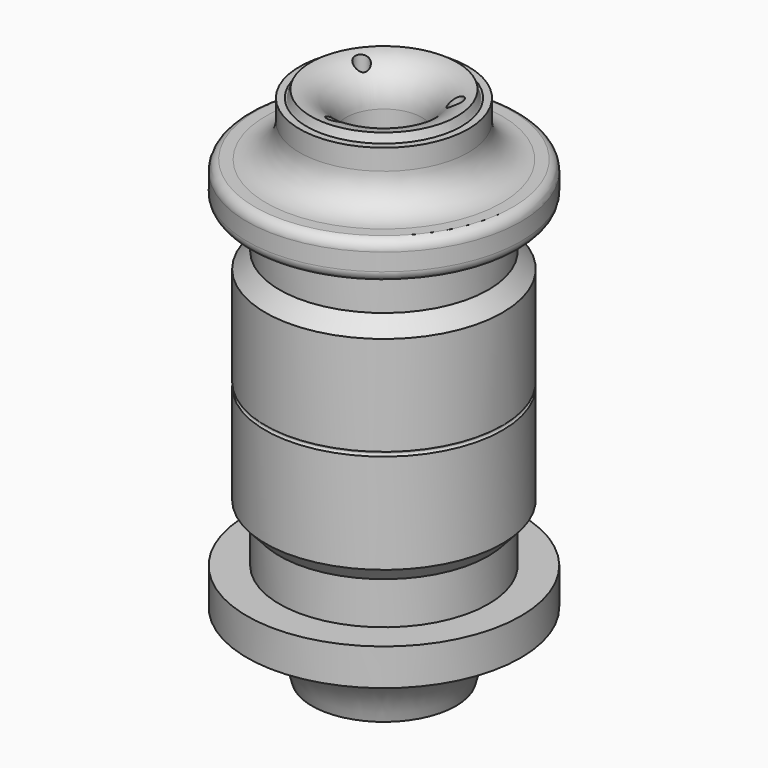
from build123d import *

# Parameters (mm, degrees)
F2_R     = 0.9926331533
F3_DEPTH = 76.962


# Not quite as in the source:
# - a fillet or chamfer that OpenCascade refuses, or shapes differently, is made with other operations: its cross-section is extruded or revolved along the edge and cut away or added


with BuildPart() as f1:
    # F0 (on Front) → F1 (revolve)
    with BuildSketch(Plane.XZ):
        with BuildLine():
            Line((5.1929587498, 60.6806613505), (5.1929587498, -10.0974142551))
            Line((5.1929587498, -10.0974142551), (9.8089184612, -10.0974142551))
            ThreePointArc((9.8089184612, -10.0974142551), (12.909244256, -4.4172381027), (18.6561793089, -1.4424845576))
            Line((18.6561793089, -1.4424845576), (18.6561793089, 3.5581402481))
            Line((18.6561793089, 3.5581402481), (14.2325470224, 3.5581402481))
            Line((14.2325470224, 3.5581402481), (14.2325470224, 9.3280896544))
            Line((14.2325470224, 9.3280896544), (16.155866906, 11.4437416196))
            Line((16.155866906, 11.4437416196), (16.155866906, 25.0280182809))
            ThreePointArc((16.155866906, 25.0280182809), (15.9726518478, 25.3139212728), (16.155866906, 25.5998242646))
            Line((16.155866906, 25.5998242646), (16.155866906, 39.1395054758))
            Line((16.155866906, 39.1395054758), (14.2325470224, 41.2551574409))
            Line((14.2325470224, 41.2551574409), (14.2325470224, 45.5512719705))
            ThreePointArc((14.2325470224, 45.5512719705), (14.6642232635, 46.5934306062), (15.7063818992, 47.0251068473))
            Line((15.7063818992, 47.0251068473), (17.1823444321, 47.0251068473))
            ThreePointArc((17.1823444321, 47.0251068473), (18.2245030678, 47.4567830884), (18.6561793089, 48.4989417241))
            Line((18.6561793089, 48.4989417241), (18.6561793089, 50.8594763109))
            ThreePointArc((18.6561793089, 50.8594763109), (18.3597063527, 51.7460473189), (17.5895630082, 52.2759374913))
            Line((17.5895630082, 52.2759374913), (16.0549388054, 52.2759374913))
            ThreePointArc((16.0549388054, 52.2759374913), (12.8346842963, 53.6098105832), (11.5008112043, 56.8300650923))
            Line((11.5008112043, 56.8300650923), (11.5008112043, 59.6561431885))
            Line((11.5008112043, 59.6561431885), (10.5512943119, 59.6561431885))
            add(Edge.make_bspline(
                [(9.9622784182, 60.6806613505), (10.0165205284, 60.4888391389), (10.1159642473, 60.1371656141), (10.2252415949, 59.8021463565), (10.3550447499, 59.4296037744), (10.4923000256, 59.5379966019), (10.5308172917, 59.6151343012), (10.5512943119, 59.6561431885)],
                knots=[0, 0, 0, 0, 0.2849514983, 0.5224102931, 0.7343274754, 0.8587599224, 1, 1, 1, 1], degree=3))
            Line((9.9622784182, 60.6806613505), (9.8089184612, 60.6806613505))
            Line((9.8089184612, 60.6806613505), (5.1929587498, 60.6806613505))
        make_face()
    revolve(axis=Axis((0, 0, 0.7693264633), (0, 0, -1)))

    # F2 (on face) → F3 (cut)
    with BuildSketch(Plane.XY.offset(60.6806613505)):
        with Locations((-6.5063127582, 4.3251969566)):
            Circle(F2_R)
        with Locations((6.9988868199, 3.4720336553)):
            Circle(F2_R)
        with Locations((-0.4925740617, -7.7972306119)):
            Circle(F2_R)
    extrude(amount=-F3_DEPTH, mode=Mode.SUBTRACT)

    # F4: fillet of radius 5.08 on 1 edges, made by hand

    # F4_s1 → F4_t2 (revolve, cut)
    with BuildSketch(Plane.XZ):
        with BuildLine():
            ThreePointArc((9.9622784182, 60.6806613505), (6.5726441629, 59.0906980139), (5.1929587498, 55.6101704737))
            Line((5.1929587498, 55.6101704737), (5.1929587498, 60.6806613505))
            Line((5.1929587498, 60.6806613505), (9.9622784182, 60.6806613505))
        make_face()
    revolve(axis=Axis((0, 0, 60.6806613505), (0, 0, -1)), mode=Mode.SUBTRACT)


solid = f1.part
